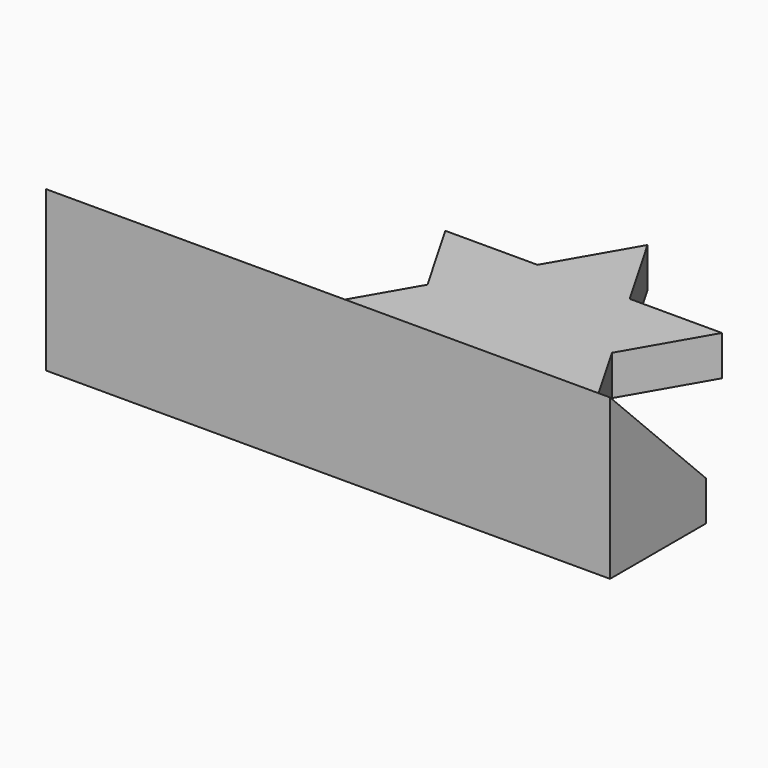
from build123d import *

# Parameters (mm, degrees)
F1_DEPTH     = 101.6
F2_DEPTH     = 25.4
F3_T4_DEPTH  = 750.6555783885
F3_T11_DEPTH = 750.6555783885
F3_T17_DEPTH = 750.6555783885
F3_T24_DEPTH = 750.6555783885
F5_TEXT_SIZE = 60.2297147092
F6_DEPTH     = 7.62


# Not quite as in the source:
# - a fillet or chamfer that OpenCascade refuses, or shapes differently, is made with other operations: its cross-section is extruded or revolved along the edge and cut away or added
# - Text() gives the source's letters only with a copy of the font that has no kerning and outlines rounded to 1/6400 em; it was checked with that copy


with BuildPart() as f1:
    # F0 (on Top) → F1 (new body)
    with BuildSketch(Plane.XY):
        Polygon((0, -101.6), (-14.6646968374, -76.2), (-179.3655455112, -76.2), (-179.3655455112, -152.4), (179.3655455112, -152.4), (179.3655455112, -76.2), (14.6646968374, -76.2), align=None)
        Polygon((14.6646968374, -76.2), (-14.6646968374, -76.2), (0, -101.6), align=None)
    extrude(amount=F1_DEPTH)

    # F0 (on Top) → F2 (join)
    with BuildSketch(Plane.XY):
        Polygon((0, 101.6), (-29.3293936748, 50.8), (29.3293936748, 50.8), align=None)
        Polygon((-29.3293936748, 50.8), (-87.9881810245, 50.8), (-58.6587873497, 0), align=None)
        Polygon((29.3293936748, 50.8), (-29.3293936748, 50.8), (-58.6587873497, 0), (-29.3293936748, -50.8), (29.3293936748, -50.8), (58.6587873497, 0), align=None)
        Polygon((-29.3293936748, -50.8), (-58.6587873497, 0), (-87.9881810245, -50.8), align=None)
        Polygon((29.3293936748, -50.8), (-29.3293936748, -50.8), (-14.6646968374, -76.2), (14.6646968374, -76.2), align=None)
        Polygon((87.9881810245, -50.8), (58.6587873497, 0), (29.3293936748, -50.8), align=None)
        Polygon((87.9881810245, 50.8), (29.3293936748, 50.8), (58.6587873497, 0), align=None)
    extrude(amount=F2_DEPTH)

    # F3: chamfer of 76.2 on 1 edges, made by hand


with BuildPart() as f3_tool2:
    # F3_s3 → F3_t4 (new body)
    with BuildSketch(Plane.YZ.offset(375.3277891942)):
        Polygon((-76.2, 25.4), (-152.4, 101.6), (-76.2, 101.6), align=None)
    extrude(amount=-F3_T4_DEPTH)

    split(bisect_by=Plane(origin=(43.9940905122, -25.4, 0), x_dir=(0, 0, 1), z_dir=(0.8660254038, -0.5, 0)), keep=Keep.TOP)

    split(bisect_by=Plane.XY.offset(25.4), keep=Keep.TOP)

    split(bisect_by=Plane(origin=(-43.9940905122, -25.4, 0), x_dir=(0, 0, 1), z_dir=(0.8660254038, 0.5, 0)), keep=Keep.TOP)


with BuildPart() as f1_1:
    add(f1.part)

    # F3_t1: cut F3_tool2
    add(f3_tool2.part, mode=Mode.SUBTRACT)


with BuildPart() as f3_tool9:
    # F3_s10 → F3_t11 (new body)
    with BuildSketch(Plane.YZ.offset(375.3277891942)):
        Polygon((-76.2, 25.4), (-152.4, 101.6), (-76.2, 101.6), align=None)
    extrude(amount=-F3_T11_DEPTH)

    split(bisect_by=Plane(origin=(43.9940905122, -25.4, 0), x_dir=(0, 0, 1), z_dir=(0.8660254038, -0.5, 0)), keep=Keep.TOP)

    split(bisect_by=Plane(origin=(-43.9940905122, -25.4, 0), x_dir=(0, 0, 1), z_dir=(-0.8660254038, -0.5, 0)), keep=Keep.TOP)


with BuildPart() as f1_2:
    add(f1_1.part)

    # F3_t8: cut F3_tool9
    add(f3_tool9.part, mode=Mode.SUBTRACT)


with BuildPart() as f3_tool15:
    # F3_s16 → F3_t17 (new body)
    with BuildSketch(Plane.YZ.offset(375.3277891942)):
        Polygon((-76.2, 25.4), (-152.4, 101.6), (-76.2, 101.6), align=None)
    extrude(amount=-F3_T17_DEPTH)

    split(bisect_by=Plane(origin=(43.9940905122, -25.4, 0), x_dir=(0, 0, 1), z_dir=(-0.8660254038, 0.5, 0)), keep=Keep.TOP)

    split(bisect_by=Plane.XY.offset(25.4), keep=Keep.TOP)

    split(bisect_by=Plane(origin=(-43.9940905122, -25.4, 0), x_dir=(0, 0, 1), z_dir=(0.8660254038, 0.5, 0)), keep=Keep.TOP)


with BuildPart() as f1_3:
    add(f1_2.part)

    # F3_t14: cut F3_tool15
    add(f3_tool15.part, mode=Mode.SUBTRACT)


with BuildPart() as f3_tool22:
    # F3_s23 → F3_t24 (new body)
    with BuildSketch(Plane.YZ.offset(375.3277891942)):
        Polygon((-76.2, 25.4), (-152.4, 101.6), (-76.2, 101.6), align=None)
    extrude(amount=-F3_T24_DEPTH)

    split(bisect_by=Plane(origin=(43.9940905122, -25.4, 0), x_dir=(0, 0, 1), z_dir=(-0.8660254038, 0.5, 0)), keep=Keep.TOP)

    split(bisect_by=Plane.XY.offset(25.4), keep=Keep.TOP)

    split(bisect_by=Plane(origin=(-43.9940905122, -25.4, 0), x_dir=(0, 0, 1), z_dir=(-0.8660254038, -0.5, 0)), keep=Keep.TOP)


with BuildPart() as f1_4:
    add(f1_3.part)

    # F3_t21: cut F3_tool22
    add(f3_tool22.part, mode=Mode.SUBTRACT)

    # F5 (on offset) → F6 (cut)
    with BuildSketch(Plane(origin=(0, -25.4, -25.4), x_dir=(-1, 0, 0), z_dir=(0, 0.7071067812, 0.7071067812))):
        with Locations(Location((152.4415455112, 144.504025477), (0, 0, -180))):
            Text('David Levy', F5_TEXT_SIZE, font='Open Sans', text_align=(TextAlign.LEFT, TextAlign.BOTTOM))
    extrude(amount=-F6_DEPTH, mode=Mode.SUBTRACT)


solid = f1_4.part
